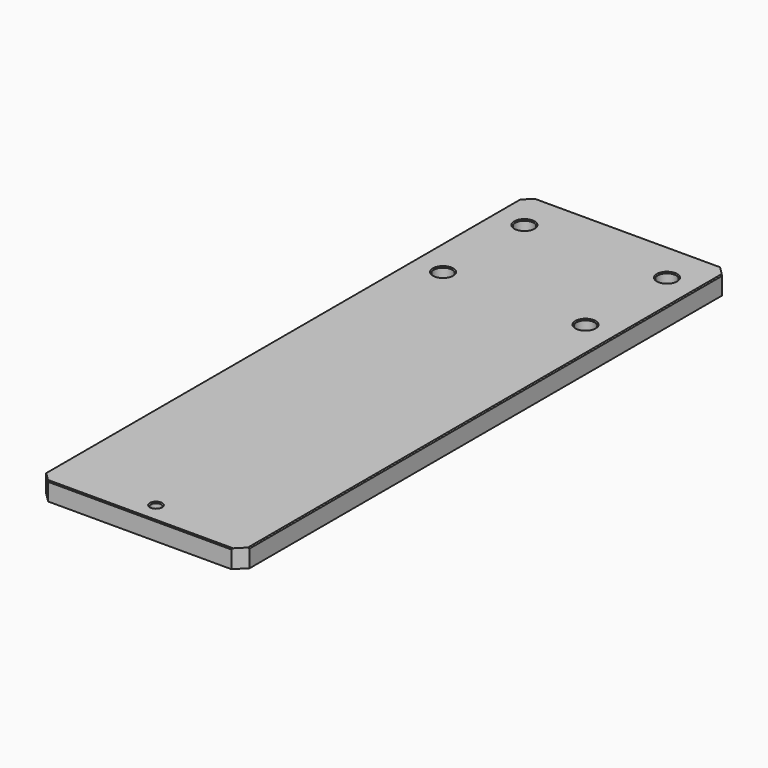
from build123d import *

# Parameters (mm, degrees)
F0_W        = 100
F0_H        = 300
F1_DEPTH    = 9
F3_D        = 9
F5_D        = 5
F6_SIZE     = 0.5
F7_T1_DEPTH = 34.2168298797


# Not quite as in the source:
# - a fillet or chamfer that OpenCascade refuses, or shapes differently, is made with other operations: its cross-section is extruded or revolved along the edge and cut away or added


with BuildPart() as f1:
    # F0 (on Top) → F1 (new body)
    with BuildSketch(Plane.XY):
        with Locations((-50, 150)):
            Rectangle(F0_W, F0_H)
    extrude(amount=F1_DEPTH)

    # F3 (through all)
    with Locations(Plane.XY.offset(9)):
        with Locations((-85, 280), (-15, 280), (-15, 230), (-85, 230)):
            Hole(F3_D / 2)

    # F5 (through all)
    with Locations(Plane.XY.offset(9)):
        with Locations((-50, 10)):
            Hole(F5_D / 2)

    # F6
    f6_edges = [f1.edges().sort_by_distance(p)[0] for p in [
        (-50, 0, 9),
        (-100, 150, 9),
        (0, 150, 9),
        (-50, 300, 9),
        (-52.5, 10, 9),
        (-89.5, 230, 9),
        (-89.5, 280, 9),
        (-19.5, 230, 9),
        (-19.5, 280, 9),
        (-52.5, 10, 0),
    ]]
    chamfer(f6_edges, length=F6_SIZE)

    # F7: chamfer of 5 on 4 edges, made by hand

    # F7_s2 → F7_t1 (cut)
    with BuildSketch(Plane.XY.offset(-12.8584149398)):
        Polygon((-95, 0), (-100, 5), (-100, 0), align=None)
        Polygon((-5, 0), (0, 5), (0, 0), align=None)
        Polygon((-100, 295), (-95, 300), (-100, 300), align=None)
        Polygon((0, 295), (-5, 300), (0, 300), align=None)
    extrude(amount=F7_T1_DEPTH, mode=Mode.SUBTRACT)


solid = f1.part
